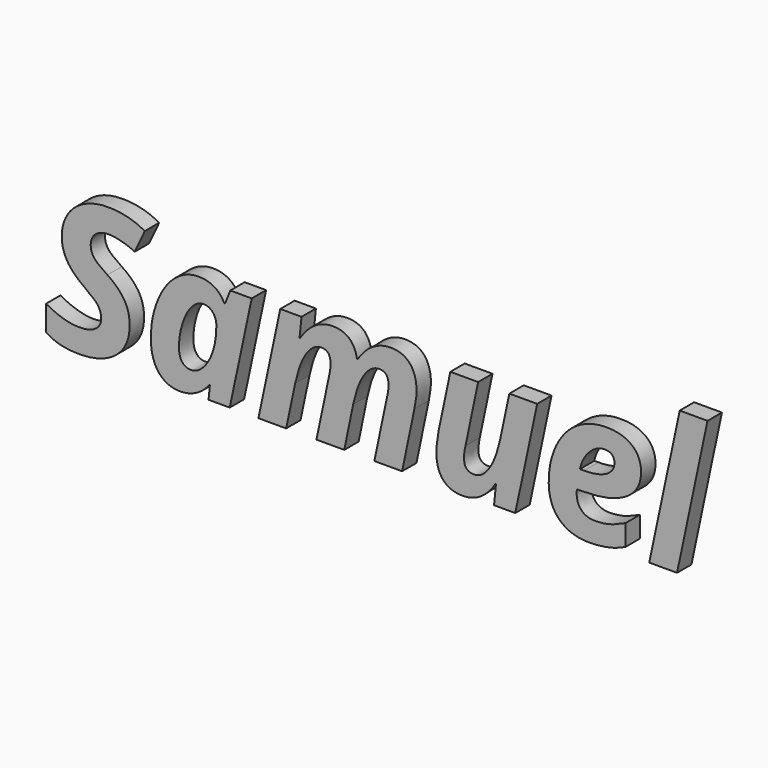
from build123d import *

# Parameters (mm, degrees)
F0_TEXT_SIZE = 53.4329265873
F1_DEPTH     = 5.08


# Not quite as in the source:
# - Text() gives the source's letters only with a copy of the font that has no kerning and outlines rounded to 1/6400 em; it was checked with that copy


with BuildPart() as f1:
    # F0 (on Front) → F1 (new body)
    with BuildSketch(Plane.XZ):
        with Locations((-65.7921954989, 3.9958534762)):
            Text('Samuel', F0_TEXT_SIZE, font='Open Sans', font_style=FontStyle.BOLDITALIC, text_align=(TextAlign.LEFT, TextAlign.BOTTOM))
    extrude(amount=F1_DEPTH)


solid = f1.part
